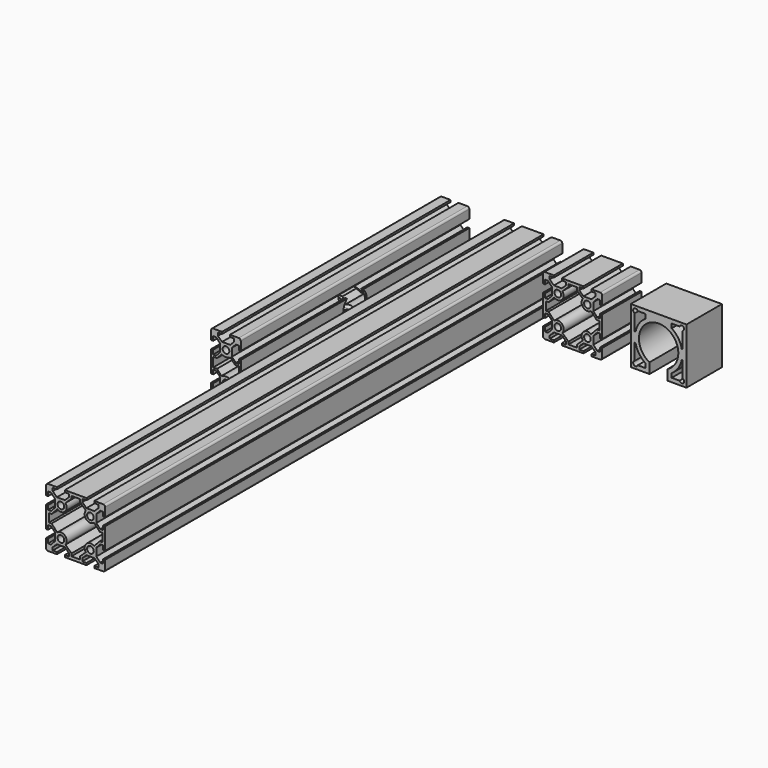
from build123d import *

# Parameters (mm, degrees)
F0_R     = 3.4
F1_DEPTH = 580
F2_DEPTH = 50
F3_DEPTH = 290
F5_DEPTH = 30
F6_DEPTH = 45


# Not quite as in the source:
# - ends of sketch curves that miss each other by under 0.0002 mm in the source are joined


with BuildPart() as f1:
    # F0 (on Front) → F1 (new body)
    with BuildSketch(Plane.XZ):
        with BuildLine():
            Line((-19, 30), (-28, 30))
            ThreePointArc((-28, 30), (-29.4142135624, 29.4142135624), (-30, 28))
            Line((-30, 28), (-30, 19))
            Line((-30, 19), (-28, 19))
            Line((-28, 19), (-28, 23.25))
            Line((-28, 23.25), (-25, 23.25))
            Line((-25, 23.25), (-21, 19))
            Line((-21, 19), (-21, 11))
            Line((-21, 11), (-25, 6.75))
            Line((-25, 6.75), (-28, 6.75))
            Line((-28, 6.75), (-28, 11))
            Line((-28, 11), (-30, 11))
            Line((-30, 11), (-30, -11))
            Line((-30, -11), (-28, -11))
            Line((-28, -11), (-28, -6.75))
            Line((-28, -6.75), (-25, -6.75))
            Line((-25, -6.75), (-21, -11))
            Line((-21, -11), (-21, -19))
            Line((-21, -19), (-25, -23.25))
            Line((-25, -23.25), (-28, -23.25))
            Line((-28, -23.25), (-28, -19))
            Line((-28, -19), (-30, -19))
            Line((-30, -19), (-30, -28))
            ThreePointArc((-30, -28), (-29.4142135624, -29.4142135624), (-28, -30))
            Line((-28, -30), (-19, -30))
            Line((-19, -30), (-19, -28))
            Line((-19, -28), (-23.25, -28))
            Line((-23.25, -28), (-23.25, -25))
            Line((-23.25, -25), (-19, -21))
            Line((-19, -21), (-10.9999906868, -21))
            Line((-10.9999906868, -21), (-6.7499906868, -25))
            Line((-6.7499906868, -25), (-6.7499906868, -28))
            Line((-6.7499906868, -28), (-10.9999906868, -28))
            Line((-10.9999906868, -28), (-10.9999906868, -30))
            Line((-10.9999906868, -30), (10.9999906868, -30))
            Line((10.9999906868, -30), (10.9999906868, -28))
            Line((10.9999906868, -28), (6.7499906868, -28))
            Line((6.7499906868, -28), (6.7499906868, -25))
            Line((6.7499906868, -25), (10.9999906868, -21))
            Line((10.9999906868, -21), (19, -21))
            Line((19, -21), (23.25, -25))
            Line((23.25, -25), (23.25, -28))
            Line((23.25, -28), (19, -28))
            Line((19, -28), (19, -30))
            Line((19, -30), (28, -30))
            ThreePointArc((28, -30), (29.4142135624, -29.4142135624), (30, -28))
            Line((30, -28), (30, -19))
            Line((30, -19), (28, -19))
            Line((28, -19), (28, -23.25))
            Line((28, -23.25), (25, -23.25))
            Line((25, -23.25), (21, -19))
            Line((21, -19), (21, -11))
            Line((21, -11), (25, -6.75))
            Line((25, -6.75), (28, -6.75))
            Line((28, -6.75), (28, -11))
            Line((28, -11), (30, -11))
            Line((30, -11), (30, 11))
            Line((30, 11), (28, 11))
            Line((28, 11), (28, 6.75))
            Line((28, 6.75), (25, 6.75))
            Line((25, 6.75), (21, 11))
            Line((21, 11), (21, 19))
            Line((21, 19), (25, 23.25))
            Line((25, 23.25), (28, 23.25))
            Line((28, 23.25), (28, 19))
            Line((28, 19), (30, 19))
            Line((30, 19), (30, 28))
            ThreePointArc((30, 28), (29.4142135624, 29.4142135624), (28, 30))
            Line((28, 30), (19, 30))
            Line((19, 30), (19, 28))
            Line((19, 28), (23.25, 28))
            Line((23.25, 28), (23.25, 25))
            Line((23.25, 25), (19, 21))
            Line((19, 21), (10.9999906868, 21))
            Line((10.9999906868, 21), (6.7499906868, 25))
            Line((6.7499906868, 25), (6.7499906868, 28))
            Line((6.7499906868, 28), (10.9999906868, 28))
            Line((10.9999906868, 28), (10.9999906868, 30))
            Line((10.9999906868, 30), (-10.9999906868, 30))
            Line((-10.9999906868, 30), (-10.9999906868, 28))
            Line((-10.9999906868, 28), (-6.7499906868, 28))
            Line((-6.7499906868, 28), (-6.7499906868, 25))
            Line((-6.7499906868, 25), (-10.9999906868, 21))
            Line((-10.9999906868, 21), (-19, 21))
            Line((-19, 21), (-23.25, 25))
            Line((-23.25, 25), (-23.25, 28))
            Line((-23.25, 28), (-19, 28))
            Line((-19, 28), (-19, 30))
        make_face()
        with Locations((-14.9999953434, -15)):
            Circle(F0_R, mode=Mode.SUBTRACT)
        with Locations((15.0000046566, -15)):
            Circle(F0_R, mode=Mode.SUBTRACT)
        with BuildLine():
            Line((-4.2499906868, 24.4029052556), (-4.2499906868, 27))
            Line((-4.2499906868, 27), (4.2499906868, 27))
            Line((4.2499906868, 27), (4.2499906868, 24.4029052556))
            Line((4.2499906868, 24.4029052556), (10.3822546259, 18.6313627246))
            ThreePointArc((10.3822546259, 18.6313627246), (10.8738554582, 10.8328944166), (18.6752136797, 10.3895105781))
            Line((18.6752136797, 10.3895105781), (24.4467562106, 4.2572466389))
            Line((24.4467562106, 4.2572466389), (27.0438509551, 4.2572466389))
            Line((27.0438509551, 4.2572466389), (27.0438509551, -4.2427347346))
            Line((27.0438509551, -4.2427347346), (24.4467562106, -4.2427347346))
            Line((24.4467562106, -4.2427347346), (18.6752136797, -10.3749986738))
            ThreePointArc((18.6752136797, -10.3749986738), (10.8720356126, -10.830274432), (10.3822546259, -18.6313627246))
            Line((10.3822546259, -18.6313627246), (4.2499906868, -24.4029052556))
            Line((4.2499906868, -24.4029052556), (4.2499906868, -27))
            Line((4.2499906868, -27), (-4.2499906868, -27))
            Line((-4.2499906868, -27), (-4.2499906868, -24.4029052556))
            Line((-4.2499906868, -24.4029052556), (-10.3822546259, -18.6313627246))
            ThreePointArc((-10.3822546259, -18.6313627246), (-10.7897356908, -10.7476097291), (-18.6752136797, -10.3749986738))
            Line((-18.6752136797, -10.3749986738), (-24.4467562106, -4.2427347346))
            Line((-24.4467562106, -4.2427347346), (-27.0438509551, -4.2427347346))
            Line((-27.0438509551, -4.2427347346), (-27.0438509551, 4.2572466389))
            Line((-27.0438509551, 4.2572466389), (-24.4467562106, 4.2572466389))
            Line((-24.4467562106, 4.2572466389), (-18.6752136797, 10.3895105781))
            ThreePointArc((-18.6752136797, 10.3895105781), (-10.8492567486, 10.8081431729), (-10.3822546259, 18.6313627246))
            Line((-10.3822546259, 18.6313627246), (-4.2499906868, 24.4029052556))
        make_face(mode=Mode.SUBTRACT)
        with Locations((-14.9999953434, 15)):
            Circle(F0_R, mode=Mode.SUBTRACT)
        with Locations((15.0000046566, 15)):
            Circle(F0_R, mode=Mode.SUBTRACT)
    extrude(amount=F1_DEPTH)


with BuildPart() as f2:
    # F0 (on Front) → F2 (new body)
    with BuildSketch(Plane.XZ):
        with BuildLine():
            Line((61.5000092089, 30), (52.5000092089, 30))
            ThreePointArc((52.5000092089, 30), (51.0857956465, 29.4142135624), (50.5000092089, 28))
            Line((50.5000092089, 28), (50.5000092089, 19))
            Line((50.5000092089, 19), (52.5000092089, 19))
            Line((52.5000092089, 19), (52.5000092089, 23.25))
            Line((52.5000092089, 23.25), (55.5000092089, 23.25))
            Line((55.5000092089, 23.25), (59.5000092089, 19))
            Line((59.5000092089, 19), (59.5000092089, 11))
            Line((59.5000092089, 11), (55.5000092089, 6.75))
            Line((55.5000092089, 6.75), (52.5000092089, 6.75))
            Line((52.5000092089, 6.75), (52.5000092089, 11))
            Line((52.5000092089, 11), (50.5000092089, 11))
            Line((50.5000092089, 11), (50.5000092089, -11))
            Line((50.5000092089, -11), (52.5000092089, -11))
            Line((52.5000092089, -11), (52.5000092089, -6.75))
            Line((52.5000092089, -6.75), (55.5000092089, -6.75))
            Line((55.5000092089, -6.75), (59.5000092089, -11))
            Line((59.5000092089, -11), (59.5000092089, -19))
            Line((59.5000092089, -19), (55.5000092089, -23.25))
            Line((55.5000092089, -23.25), (52.5000092089, -23.25))
            Line((52.5000092089, -23.25), (52.5000092089, -19))
            Line((52.5000092089, -19), (50.5000092089, -19))
            Line((50.5000092089, -19), (50.5000092089, -28))
            ThreePointArc((50.5000092089, -28), (51.0857956465, -29.4142135624), (52.5000092089, -30))
            Line((52.5000092089, -30), (61.5000092089, -30))
            Line((61.5000092089, -30), (61.5000092089, -28))
            Line((61.5000092089, -28), (57.2500092089, -28))
            Line((57.2500092089, -28), (57.2500092089, -25))
            Line((57.2500092089, -25), (61.5000092089, -21))
            Line((61.5000092089, -21), (69.5000185221, -21))
            Line((69.5000185221, -21), (73.7500185221, -25))
            Line((73.7500185221, -25), (73.7500185221, -28))
            Line((73.7500185221, -28), (69.5000185221, -28))
            Line((69.5000185221, -28), (69.5000185221, -30))
            Line((69.5000185221, -30), (91.4999998957, -30))
            Line((91.4999998957, -30), (91.4999998957, -28))
            Line((91.4999998957, -28), (87.2499998957, -28))
            Line((87.2499998957, -28), (87.2499998957, -25))
            Line((87.2499998957, -25), (91.4999998957, -21))
            Line((91.4999998957, -21), (99.5000092089, -21))
            Line((99.5000092089, -21), (103.7500092089, -25))
            Line((103.7500092089, -25), (103.7500092089, -28))
            Line((103.7500092089, -28), (99.5000092089, -28))
            Line((99.5000092089, -28), (99.5000092089, -30))
            Line((99.5000092089, -30), (108.5000092089, -30))
            ThreePointArc((108.5000092089, -30), (109.9142227713, -29.4142135624), (110.5000092089, -28))
            Line((110.5000092089, -28), (110.5000092089, -19))
            Line((110.5000092089, -19), (108.5000092089, -19))
            Line((108.5000092089, -19), (108.5000092089, -23.25))
            Line((108.5000092089, -23.25), (105.5000092089, -23.25))
            Line((105.5000092089, -23.25), (101.5000092089, -19))
            Line((101.5000092089, -19), (101.5000092089, -11))
            Line((101.5000092089, -11), (105.5000092089, -6.75))
            Line((105.5000092089, -6.75), (108.5000092089, -6.75))
            Line((108.5000092089, -6.75), (108.5000092089, -11))
            Line((108.5000092089, -11), (110.5000092089, -11))
            Line((110.5000092089, -11), (110.5000092089, 11))
            Line((110.5000092089, 11), (108.5000092089, 11))
            Line((108.5000092089, 11), (108.5000092089, 6.75))
            Line((108.5000092089, 6.75), (105.5000092089, 6.75))
            Line((105.5000092089, 6.75), (101.5000092089, 11))
            Line((101.5000092089, 11), (101.5000092089, 19))
            Line((101.5000092089, 19), (105.5000092089, 23.25))
            Line((105.5000092089, 23.25), (108.5000092089, 23.25))
            Line((108.5000092089, 23.25), (108.5000092089, 19))
            Line((108.5000092089, 19), (110.5000092089, 19))
            Line((110.5000092089, 19), (110.5000092089, 28))
            ThreePointArc((110.5000092089, 28), (109.9142227713, 29.4142135624), (108.5000092089, 30))
            Line((108.5000092089, 30), (99.5000092089, 30))
            Line((99.5000092089, 30), (99.5000092089, 28))
            Line((99.5000092089, 28), (103.7500092089, 28))
            Line((103.7500092089, 28), (103.7500092089, 25))
            Line((103.7500092089, 25), (99.5000092089, 21))
            Line((99.5000092089, 21), (91.4999998957, 21))
            Line((91.4999998957, 21), (87.2499998957, 25))
            Line((87.2499998957, 25), (87.2499998957, 28))
            Line((87.2499998957, 28), (91.4999998957, 28))
            Line((91.4999998957, 28), (91.4999998957, 30))
            Line((91.4999998957, 30), (69.5000185221, 30))
            Line((69.5000185221, 30), (69.5000185221, 28))
            Line((69.5000185221, 28), (73.7500185221, 28))
            Line((73.7500185221, 28), (73.7500185221, 25))
            Line((73.7500185221, 25), (69.5000185221, 21))
            Line((69.5000185221, 21), (61.5000092089, 21))
            Line((61.5000092089, 21), (57.2500092089, 25))
            Line((57.2500092089, 25), (57.2500092089, 28))
            Line((57.2500092089, 28), (61.5000092089, 28))
            Line((61.5000092089, 28), (61.5000092089, 30))
        make_face()
        with Locations((65.5000138655, -15)):
            Circle(F0_R, mode=Mode.SUBTRACT)
        with Locations((95.5000138655, -15)):
            Circle(F0_R, mode=Mode.SUBTRACT)
        with BuildLine():
            Line((76.2500185221, 24.4029052556), (76.2500185221, 27))
            Line((76.2500185221, 27), (84.7499998957, 27))
            Line((84.7499998957, 27), (84.7499998957, 24.4029052556))
            Line((84.7499998957, 24.4029052556), (90.8822638349, 18.6313627246))
            ThreePointArc((90.8822638349, 18.6313627246), (91.3738646671, 10.8328944166), (99.1752228886, 10.3895105781))
            Line((99.1752228886, 10.3895105781), (104.9467654196, 4.2572466389))
            Line((104.9467654196, 4.2572466389), (107.543860164, 4.2572466389))
            Line((107.543860164, 4.2572466389), (107.543860164, -4.2427347346))
            Line((107.543860164, -4.2427347346), (104.9467654196, -4.2427347346))
            Line((104.9467654196, -4.2427347346), (99.1752228886, -10.3749986738))
            ThreePointArc((99.1752228886, -10.3749986738), (91.3720448215, -10.830274432), (90.8822638349, -18.6313627246))
            Line((90.8822638349, -18.6313627246), (84.7499998957, -24.4029052556))
            Line((84.7499998957, -24.4029052556), (84.7499998957, -27))
            Line((84.7499998957, -27), (76.2500185221, -27))
            Line((76.2500185221, -27), (76.2500185221, -24.4029052556))
            Line((76.2500185221, -24.4029052556), (70.117754583, -18.6313627246))
            ThreePointArc((70.117754583, -18.6313627246), (69.7102735181, -10.7476097291), (61.8247955292, -10.3749986738))
            Line((61.8247955292, -10.3749986738), (56.0532529983, -4.2427347346))
            Line((56.0532529983, -4.2427347346), (53.4561582538, -4.2427347346))
            Line((53.4561582538, -4.2427347346), (53.4561582538, 4.2572466389))
            Line((53.4561582538, 4.2572466389), (56.0532529983, 4.2572466389))
            Line((56.0532529983, 4.2572466389), (61.8247955292, 10.3895105781))
            ThreePointArc((61.8247955292, 10.3895105781), (69.6507524603, 10.8081431729), (70.117754583, 18.6313627246))
            Line((70.117754583, 18.6313627246), (76.2500185221, 24.4029052556))
        make_face(mode=Mode.SUBTRACT)
        with Locations((65.5000138655, 15)):
            Circle(F0_R, mode=Mode.SUBTRACT)
        with Locations((95.5000138655, 15)):
            Circle(F0_R, mode=Mode.SUBTRACT)
    extrude(amount=F2_DEPTH)


with BuildPart() as f3:
    # F0 (on Front) → F3 (new body)
    with BuildSketch(Plane.XZ):
        with BuildLine():
            Line((-83.3785533309, 30), (-92.3785533309, 30))
            ThreePointArc((-92.3785533309, 30), (-93.7927668933, 29.4142135624), (-94.3785533309, 28))
            Line((-94.3785533309, 28), (-94.3785533309, 19))
            Line((-94.3785533309, 19), (-92.3785533309, 19))
            Line((-92.3785533309, 19), (-92.3785533309, 23.25))
            Line((-92.3785533309, 23.25), (-89.3785533309, 23.25))
            Line((-89.3785533309, 23.25), (-85.3785533309, 19))
            Line((-85.3785533309, 19), (-85.3785533309, 11))
            Line((-85.3785533309, 11), (-89.3785533309, 6.75))
            Line((-89.3785533309, 6.75), (-92.3785533309, 6.75))
            Line((-92.3785533309, 6.75), (-92.3785533309, 11))
            Line((-92.3785533309, 11), (-94.3785533309, 11))
            Line((-94.3785533309, 11), (-94.3785533309, -11))
            Line((-94.3785533309, -11), (-92.3785533309, -11))
            Line((-92.3785533309, -11), (-92.3785533309, -6.75))
            Line((-92.3785533309, -6.75), (-89.3785533309, -6.75))
            Line((-89.3785533309, -6.75), (-85.3785533309, -11))
            Line((-85.3785533309, -11), (-85.3785533309, -19))
            Line((-85.3785533309, -19), (-89.3785533309, -23.25))
            Line((-89.3785533309, -23.25), (-92.3785533309, -23.25))
            Line((-92.3785533309, -23.25), (-92.3785533309, -19))
            Line((-92.3785533309, -19), (-94.3785533309, -19))
            Line((-94.3785533309, -19), (-94.3785533309, -28))
            ThreePointArc((-94.3785533309, -28), (-93.7927668933, -29.4142135624), (-92.3785533309, -30))
            Line((-92.3785533309, -30), (-83.3785533309, -30))
            Line((-83.3785533309, -30), (-83.3785533309, -28))
            Line((-83.3785533309, -28), (-87.6285533309, -28))
            Line((-87.6285533309, -28), (-87.6285533309, -25))
            Line((-87.6285533309, -25), (-83.3785533309, -21))
            Line((-83.3785533309, -21), (-75.0943720341, -21))
            Line((-75.0943720341, -21), (-71.1285533309, -25))
            Line((-71.1285533309, -25), (-71.1285533309, -28))
            Line((-71.1285533309, -28), (-75.3785533309, -28))
            Line((-75.3785533309, -28), (-75.3785533309, -30))
            Line((-75.3785533309, -30), (-66.3785533309, -30))
            ThreePointArc((-66.3785533309, -30), (-64.9643397685, -29.4142135624), (-64.3785533309, -28))
            Line((-64.3785533309, -28), (-64.3785533309, -19))
            Line((-64.3785533309, -19), (-66.3785533309, -19))
            Line((-66.3785533309, -19), (-66.3785533309, -23.25))
            Line((-66.3785533309, -23.25), (-69.3785533309, -23.25))
            Line((-69.3785533309, -23.25), (-73.3785533309, -19))
            Line((-73.3785533309, -19), (-73.3785533309, -11))
            Line((-73.3785533309, -11), (-69.3785533309, -6.75))
            Line((-69.3785533309, -6.75), (-66.3785533309, -6.75))
            Line((-66.3785533309, -6.75), (-66.3785533309, -11))
            Line((-66.3785533309, -11), (-64.3785533309, -11))
            Line((-64.3785533309, -11), (-64.3785533309, 11))
            Line((-64.3785533309, 11), (-66.3785533309, 11))
            Line((-66.3785533309, 11), (-66.3785533309, 6.75))
            Line((-66.3785533309, 6.75), (-69.3785533309, 6.75))
            Line((-69.3785533309, 6.75), (-73.3785533309, 11))
            Line((-73.3785533309, 11), (-73.3785533309, 19))
            Line((-73.3785533309, 19), (-69.3785533309, 23.25))
            Line((-69.3785533309, 23.25), (-66.3785533309, 23.25))
            Line((-66.3785533309, 23.25), (-66.3785533309, 19))
            Line((-66.3785533309, 19), (-64.3785533309, 19))
            Line((-64.3785533309, 19), (-64.3785533309, 28))
            ThreePointArc((-64.3785533309, 28), (-64.9643397685, 29.4142135624), (-66.3785533309, 30))
            Line((-66.3785533309, 30), (-75.3785533309, 30))
            Line((-75.3785533309, 30), (-75.3785533309, 28))
            Line((-75.3785533309, 28), (-71.1285533309, 28))
            Line((-71.1285533309, 28), (-71.1285533309, 25))
            Line((-71.1285533309, 25), (-75.0943720341, 21))
            Line((-75.0943720341, 21), (-83.3785533309, 21))
            Line((-83.3785533309, 21), (-87.6285533309, 25))
            Line((-87.6285533309, 25), (-87.6285533309, 28))
            Line((-87.6285533309, 28), (-83.3785533309, 28))
            Line((-83.3785533309, 28), (-83.3785533309, 30))
        make_face()
        with Locations((-79.3785533309, -15)):
            Circle(F0_R, mode=Mode.SUBTRACT)
        with BuildLine():
            Line((-92.3785533309, -4.75), (-92.3785533309, 4.75))
            Line((-92.3785533309, 4.75), (-88.5144079637, 4.7499998473))
            Line((-88.5144079637, 4.7499998473), (-83.9221532343, 9.6292704973))
            ThreePointArc((-83.9221532343, 9.6292704973), (-79.3785533309, 8.6971541325), (-74.8349534275, 9.6292704973))
            Line((-74.8349534275, 9.6292704973), (-70.242698698, 4.7499998473))
            Line((-70.242698698, 4.7499998473), (-66.3785533309, 4.7499998473))
            Line((-66.3785533309, 4.7499998473), (-66.3785533309, -4.75))
            Line((-66.3785533309, -4.75), (-70.242698698, -4.7499998473))
            Line((-70.242698698, -4.7499998473), (-74.8349534275, -9.6292704973))
            ThreePointArc((-74.8349534275, -9.6292704973), (-79.3785533309, -8.6971541325), (-83.9221532343, -9.6292704973))
            Line((-83.9221532343, -9.6292704973), (-88.5144079637, -4.7499998473))
            Line((-88.5144079637, -4.7499998473), (-92.3785533309, -4.75))
        make_face(mode=Mode.SUBTRACT)
        with Locations((-79.3785533309, 15)):
            Circle(F0_R, mode=Mode.SUBTRACT)
    extrude(amount=F3_DEPTH)

    # F4 (on face) → F5 (cut)
    with BuildSketch(Plane(origin=(-94.3785533309, 0, 0), x_dir=(0, -1, 0), z_dir=(-1, 0, 0))):
        with BuildLine():
            Line((134.8019609728, 11), (155.1980390272, 11))
            ThreePointArc((155.1980390272, 11), (145, 15), (134.8019609728, 11))
        make_face()
        with BuildLine():
            ThreePointArc((134.8019609728, -11), (145, -15), (155.1980390272, -11))
            Line((155.1980390272, -11), (134.8019609728, -11))
        make_face()
        with BuildLine():
            ThreePointArc((155.1980390272, -11), (158.7471921753, -6.0012254829), (160, 0))
            ThreePointArc((160, 0), (158.7471921753, 6.0012254829), (155.1980390272, 11))
            Line((155.1980390272, 11), (134.8019609728, 11))
            ThreePointArc((134.8019609728, 11), (130, 0), (134.8019609728, -11))
            Line((134.8019609728, -11), (155.1980390272, -11))
        make_face()
    extrude(amount=-F5_DEPTH, mode=Mode.SUBTRACT)


with BuildPart() as f6:
    # F0 (on Front) → F6 (new body)
    with BuildSketch(Plane.XZ):
        with BuildLine():
            Line((135.5587966444, 26.5), (135.5587966444, -30))
            Line((135.5587966444, -30), (154.5587966444, -30))
            Line((154.5587966444, -30), (154.5587966444, -19.4823856263))
            ThreePointArc((154.5587966444, -19.4823856263), (163.8087966444, 18.25), (173.0587966444, -19.4823856263))
            Line((173.0587966444, -19.4823856263), (173.0587966444, -30))
            Line((173.0587966444, -30), (192.0587966444, -30))
            Line((192.0587966444, -30), (192.0587966444, 26.5))
            Line((192.0587966444, 26.5), (135.5587966444, 26.5))
        make_face()
        with BuildLine():
            Line((139.5587966444, -22.9970300106), (139.5587966444, -6.75))
            Line((139.5587966444, -6.75), (140.3354074558, -6.75))
            ThreePointArc((140.3354074558, -6.75), (143.9723688637, -15.2598531784), (150.5587966444, -21.7609345109))
            Line((150.5587966444, -21.7609345109), (150.5587966444, -26))
            Line((150.5587966444, -26), (142.5617666338, -26))
            ThreePointArc((142.5617666338, -26), (138.6297532004, -26.9290434439), (139.5587966444, -22.9970300106))
        make_face(mode=Mode.SUBTRACT)
        with BuildLine():
            Line((185.0558266549, -26), (177.0587966444, -26))
            Line((177.0587966444, -26), (177.0587966444, -21.7609345109))
            ThreePointArc((177.0587966444, -21.7609345109), (183.645224425, -15.2598531784), (187.282185833, -6.75))
            Line((187.282185833, -6.75), (188.0587966444, -6.75))
            Line((188.0587966444, -6.75), (188.0587966444, -22.9970300106))
            ThreePointArc((188.0587966444, -22.9970300106), (188.9878400883, -26.9290434439), (185.0558266549, -26))
        make_face(mode=Mode.SUBTRACT)
        with BuildLine():
            Line((140.3354074558, 3.25), (139.5587966444, 3.25))
            Line((139.5587966444, 3.25), (139.5587966444, 19.4970300106))
            ThreePointArc((139.5587966444, 19.4970300106), (138.6297532004, 23.4290434439), (142.5617666338, 22.5))
            Line((142.5617666338, 22.5), (150.5587966444, 22.5))
            Line((150.5587966444, 22.5), (150.5587966444, 18.2609345109))
            ThreePointArc((150.5587966444, 18.2609345109), (143.9723688637, 11.7598531784), (140.3354074558, 3.25))
        make_face(mode=Mode.SUBTRACT)
        with BuildLine():
            ThreePointArc((187.282185833, 3.25), (183.645224425, 11.7598531784), (177.0587966444, 18.2609345109))
            Line((177.0587966444, 18.2609345109), (177.0587966444, 22.5))
            Line((177.0587966444, 22.5), (185.0558266549, 22.5))
            ThreePointArc((185.0558266549, 22.5), (188.9878400883, 23.4290434439), (188.0587966444, 19.4970300106))
            Line((188.0587966444, 19.4970300106), (188.0587966444, 3.25))
            Line((188.0587966444, 3.25), (187.282185833, 3.25))
        make_face(mode=Mode.SUBTRACT)
    extrude(amount=F6_DEPTH)


solid = Compound([f1.part, f2.part, f3.part, f6.part])
